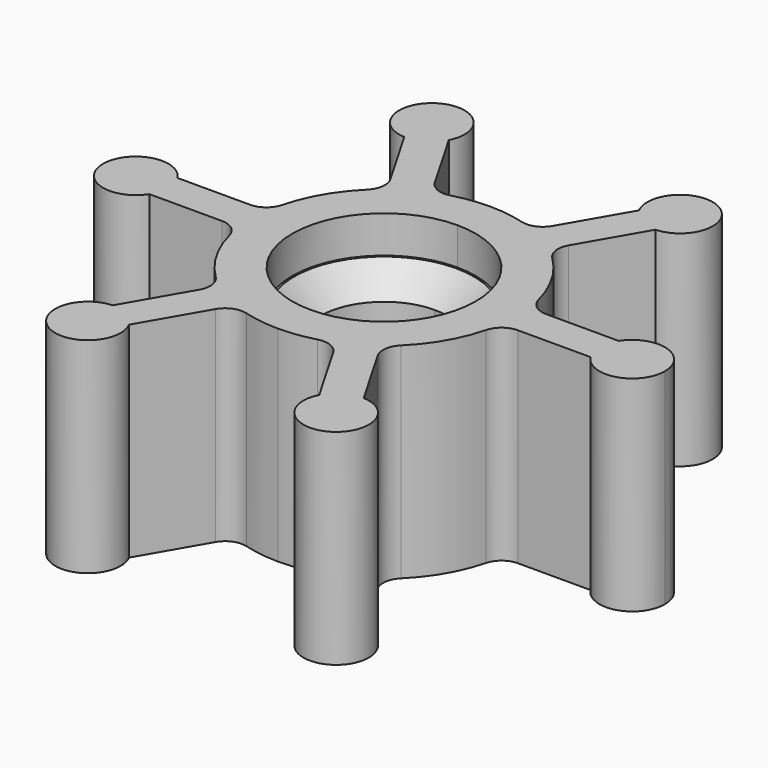
from build123d import *

# Parameters (mm, degrees)
F1_DEPTH     = 12.7508
F2_START     = 2.3114
F2_DEPTH     = 8.128
F3_R         = 1.27
F4_T4_DEPTH  = 13.1696453782
F4_S5_R      = 3.9624
F4_T6_DEPTH  = 8
F4_T15_DEPTH = 13.1696453782
F4_S16_R     = 3.9624
F4_T17_DEPTH = 8


# Not quite as in the source:
# - a fillet or chamfer that OpenCascade refuses, or shapes differently, is made with other operations: its cross-section is extruded or revolved along the edge and cut away or added
# - a feature names something its author has since deleted; it is built from what else it names


with BuildPart() as f1:
    # F0 (on Top) → F1 (new body)
    with BuildSketch(Plane.XY):
        with BuildLine():
            ThreePointArc((0, -5.7023), (-5.7023, 0), (0, 5.7023))
            Line((0, 5.7023), (0, 8.2296))
            ThreePointArc((0, 8.2296), (-1.596599089, 8.0732389726), (-3.1325279453, 7.6100975573))
            Line((-3.1325279453, 7.6100975573), (-5.9126210852, 12.4253601255))
            ThreePointArc((-5.9126210852, 12.4253601255), (-8.73125, 15.1229686136), (-7.8043669773, 11.3331601255))
            Line((-7.8043669773, 11.3331601255), (-5.0242738373, 6.5178975573))
            ThreePointArc((-5.0242738373, 6.5178975573), (-7.127042663, 4.1148), (-8.1568017826, 1.0922))
            Line((-8.1568017826, 1.0922), (-13.7169880625, 1.0922))
            ThreePointArc((-13.7169880625, 1.0922), (-17.4625, 0), (-13.7169880625, -1.0922))
            Line((-13.7169880625, -1.0922), (-8.1568017826, -1.0922))
            ThreePointArc((-8.1568017826, -1.0922), (-7.127042663, -4.1148), (-5.0242738373, -6.5178975573))
            Line((-5.0242738373, -6.5178975573), (-7.8043669773, -11.3331601255))
            ThreePointArc((-7.8043669773, -11.3331601255), (-8.73125, -15.1229686136), (-5.9126210852, -12.4253601255))
            Line((-5.9126210852, -12.4253601255), (-3.1325279453, -7.6100975573))
            ThreePointArc((-3.1325279453, -7.6100975573), (-1.596599089, -8.0732389726), (0, -8.2296))
            Line((0, -8.2296), (0, -5.7023))
        make_face()
        with BuildLine():
            ThreePointArc((0, 5.7023), (4.0321349984, 4.0321349984), (5.7023, 0))
            ThreePointArc((5.7023, 0), (4.0321349984, -4.0321349984), (0, -5.7023))
            Line((0, -5.7023), (0, -8.2296))
            ThreePointArc((0, -8.2296), (1.596599089, -8.0732389726), (3.1325279453, -7.6100975573))
            Line((3.1325279453, -7.6100975573), (5.9126210852, -12.4253601255))
            ThreePointArc((5.9126210852, -12.4253601255), (8.73125, -15.1229686136), (7.8043669773, -11.3331601255))
            Line((7.8043669773, -11.3331601255), (5.0242738373, -6.5178975573))
            ThreePointArc((5.0242738373, -6.5178975573), (7.127042663, -4.1148), (8.1568017826, -1.0922))
            Line((8.1568017826, -1.0922), (13.7169880625, -1.0922))
            ThreePointArc((13.7169880625, -1.0922), (15.9993443297, -1.9507537334), (17.4625, 0))
            ThreePointArc((17.4625, 0), (15.9993443297, 1.9507537334), (13.7169880625, 1.0922))
            Line((13.7169880625, 1.0922), (8.1568017826, 1.0922))
            ThreePointArc((8.1568017826, 1.0922), (7.127042663, 4.1148), (5.0242738373, 6.5178975573))
            Line((5.0242738373, 6.5178975573), (7.8043669773, 11.3331601255))
            ThreePointArc((7.8043669773, 11.3331601255), (8.73125, 15.1229686136), (5.9126210852, 12.4253601255))
            Line((5.9126210852, 12.4253601255), (3.1325279453, 7.6100975573))
            ThreePointArc((3.1325279453, 7.6100975573), (1.596599089, 8.0732389726), (0, 8.2296))
            Line((0, 8.2296), (0, 5.7023))
        make_face()
    extrude(amount=F1_DEPTH)

    # F0 (on Top) → F2 (join)
    with BuildSketch(Plane.XY.offset(F2_START)):
        with BuildLine():
            Line((0, 3.9624), (0, 5.7023))
            ThreePointArc((0, 5.7023), (-5.7023, 0), (0, -5.7023))
            Line((0, -5.7023), (0, -3.1496))
            Line((0, -3.1496), (-2.4042948239, -3.1496))
            ThreePointArc((-2.4042948239, -3.1496), (-3.7537040906, 1.2689835933), (0, 3.9624))
        make_face()
        with BuildLine():
            ThreePointArc((0, -5.7023), (4.0321349984, -4.0321349984), (5.7023, 0))
            ThreePointArc((5.7023, 0), (4.0321349984, 4.0321349984), (0, 5.7023))
            Line((0, 5.7023), (0, 3.9624))
            ThreePointArc((0, 3.9624), (3.7537040906, 1.2689835933), (2.4042948239, -3.1496))
            Line((2.4042948239, -3.1496), (0, -3.1496))
            Line((0, -3.1496), (0, -5.7023))
        make_face()
    extrude(amount=F2_DEPTH)

    # F3
    f3_edges = [f1.edges().sort_by_distance(p)[0] for p in [
        (-8.156802, 1.0922, 6.3754),
        (-8.156802, -1.0922, 6.3754),
        (3.132528, 7.610098, 6.3754),
        (-3.132528, 7.610098, 6.3754),
        (5.024274, 6.517898, 6.3754),
        (8.156802, 1.0922, 6.3754),
        (8.156802, -1.0922, 6.3754),
        (5.024274, -6.517898, 6.3754),
        (3.132528, -7.610098, 6.3754),
        (-3.132528, -7.610098, 6.3754),
        (-5.024274, -6.517898, 6.3754),
        (-5.024274, 6.517898, 6.3754),
    ]]
    fillet(f3_edges, radius=F3_R)

    # F4: chamfer of 1.6256 on 4 edges, made by hand


with BuildPart() as f4_tool2:
    # F4_s3 → F4_t4 (new body)
    with BuildSketch(Plane.YZ.offset(6.5848226891)):
        Polygon((-3.1496, 3.937), (-4.7752, 2.3114), (-3.1496, 2.3114), align=None)
    extrude(amount=-F4_T4_DEPTH)

    # F4_s5 → F4_t6 (intersect, symmetric)
    with BuildSketch(Plane.XY.offset(3.1)):
        Circle(F4_S5_R)
    extrude(amount=F4_T6_DEPTH, both=True, mode=Mode.INTERSECT)


with BuildPart() as f1_1:
    add(f1.part)

    # F4_t1: cut F4_tool2
    add(f4_tool2.part, mode=Mode.SUBTRACT)


with BuildPart() as f4_tool8:
    # F4_s9 → F4_t10 (revolve)
    with BuildSketch(Plane(origin=(0, 0, 0), x_dir=(0, 0, 1), z_dir=(0.7948717949, -0.6067774137, 0))):
        Polygon((3.937, 3.9624), (2.3114, 5.588), (2.3114, 3.9624), align=None)
    revolve(axis=Axis((0, 0, 2.3114), (0, 0, -1)))

    split(bisect_by=Plane(origin=(0, -3.5433, 3.5433), x_dir=(1, 0, 0), z_dir=(0, 0.7071067812, -0.7071067812)), keep=Keep.TOP)


with BuildPart() as f1_2:
    add(f1_1.part)

    # F4_t7: cut F4_tool8
    add(f4_tool8.part, mode=Mode.SUBTRACT)


with BuildPart() as f4_tool13:
    # F4_s14 → F4_t15 (new body)
    with BuildSketch(Plane.YZ.offset(6.5848226891)):
        Polygon((-4.7752, 10.4394), (-3.1496, 8.8138), (-3.1496, 10.4394), align=None)
    extrude(amount=-F4_T15_DEPTH)

    # F4_s16 → F4_t17 (intersect, symmetric)
    with BuildSketch(Plane.XY.offset(9.6)):
        Circle(F4_S16_R)
    extrude(amount=F4_T17_DEPTH, both=True, mode=Mode.INTERSECT)


with BuildPart() as f1_3:
    add(f1_2.part)

    # F4_t12: cut F4_tool13
    add(f4_tool13.part, mode=Mode.SUBTRACT)


with BuildPart() as f4_tool19:
    # F4_s20 → F4_t21 (revolve)
    with BuildSketch(Plane(origin=(0, 0, 0), x_dir=(0, 0, 1), z_dir=(0.7948717949, -0.6067774137, 0))):
        Polygon((10.4394, 5.588), (8.8138, 3.9624), (10.4394, 3.9624), align=None)
    revolve(axis=Axis((0, 0, 10.4394), (0, 0, -1)))

    split(bisect_by=Plane(origin=(0, 2.8321, 2.8321), x_dir=(1, 0, 0), z_dir=(0, 0.7071067812, 0.7071067812)), keep=Keep.TOP)


with BuildPart() as f1_4:
    add(f1_3.part)

    # F4_t18: cut F4_tool19
    add(f4_tool19.part, mode=Mode.SUBTRACT)


solid = f1_4.part
